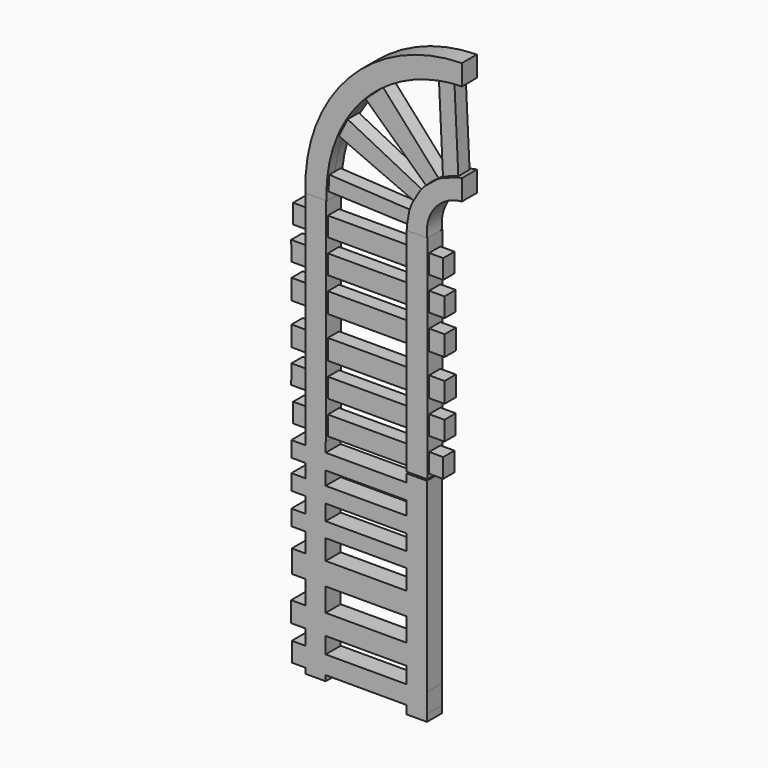
from build123d import *

# Parameters (mm, degrees)
F0_W          = 11.176
F0_H          = 7.62
F0_H_2        = 10.414
F0_H_3        = 10.414198041
F0_H_4        = 10.8981402591
F0_H_5        = 11.3893379234
F0_H_6        = 2.1167141254
F1_DEPTH      = 5.08
F1_DEPTH_BACK = 5.08
F0_W_2        = 43.688
F0_W_3        = 7.62
F0_W_4        = 8.491490941
F0_W_5        = 8.3875925946
F0_W_6        = 8.3293178785
F2_DEPTH      = 3.81
F2_DEPTH_BACK = 3.81
F4_DEPTH      = 5.08
F4_DEPTH_BACK = 5.08
F5_DEPTH      = 3.81
F5_DEPTH_BACK = 3.81
F7_W          = 43.8599754125
F7_H          = 8.4492750466
F7_W_2        = 7.6811425388
F7_H_2        = 8.4492713213
F7_H_3        = 8.4492787719
F7_W_3        = 7.454264909
F7_H_4        = 12.1605284512
F7_W_4        = 7.7864341438
F7_H_5        = 11.0083520412
F7_H_6        = 10.4579478502
F7_H_7        = 9.8724365234
F7_H_8        = 8.0819129944
F8_DEPTH      = 5.08


# Not quite as in the source:
# - a feature names something its author has since deleted; it is built from what else it names


with BuildPart() as f1:
    # F0 (on Front) → F1 (new body, two sides)
    with BuildSketch(Plane.XZ) as f1_sk:
        with Locations((-27.432, 56.4710072617)):
            Rectangle(F0_W, F0_H)
        with Locations((-27.432, 47.4540072617)):
            Rectangle(F0_W, F0_H_2)
        with Locations((-27.432, 38.4370072617)):
            Rectangle(F0_W, F0_H)
        with Locations((-27.432, 29.4199082413)):
            Rectangle(F0_W, F0_H_3)
        with Locations((-27.432, 20.4028092208)):
            Rectangle(F0_W, F0_H)
        with Locations((-27.432, 11.1437390912)):
            Rectangle(F0_W, F0_H_4)
        with Locations((-27.432, 0)):
            Rectangle(F0_W, F0_H_5)
        with Locations((-27.432, -11.1437390912)):
            Rectangle(F0_W, F0_H_4)
        with Locations((-27.432, -20.4028092208)):
            Rectangle(F0_W, F0_H)
        with Locations((-27.432, -29.4199082413)):
            Rectangle(F0_W, F0_H_3)
        with Locations((-27.432, -38.4370072617)):
            Rectangle(F0_W, F0_H)
        with Locations((-27.432, -47.4540072617)):
            Rectangle(F0_W, F0_H_2)
        with Locations((-27.432, -53.7193643245)):
            Rectangle(F0_W, F0_H_6)
    extrude(amount=F1_DEPTH)
    extrude(f1_sk.sketch, amount=-F1_DEPTH_BACK)



with BuildPart() as f1b:
    # F0 (on Front) → F1, piece 2 (new body, two sides)
    with BuildSketch(Plane.XZ) as f1_2_sk:
        with Locations((27.432, -47.4540072617)):
            Rectangle(F0_W, F0_H_2)
        with Locations((27.432, -38.4370072617)):
            Rectangle(F0_W, F0_H)
        with Locations((27.432, -29.4199082413)):
            Rectangle(F0_W, F0_H_3)
        with Locations((27.432, -20.4028092208)):
            Rectangle(F0_W, F0_H)
        with Locations((27.432, -11.1437390912)):
            Rectangle(F0_W, F0_H_4)
        with Locations((27.432, 0)):
            Rectangle(F0_W, F0_H_5)
        with Locations((27.432, 11.1437390912)):
            Rectangle(F0_W, F0_H_4)
        with Locations((27.432, 20.4028092208)):
            Rectangle(F0_W, F0_H)
        with Locations((27.432, 29.4199082413)):
            Rectangle(F0_W, F0_H_3)
        with Locations((27.432, 38.4370072617)):
            Rectangle(F0_W, F0_H)
        with Locations((27.432, 47.4540072617)):
            Rectangle(F0_W, F0_H_2)
        with Locations((27.432, 56.4710072617)):
            Rectangle(F0_W, F0_H)
        with Locations((27.432, -53.7193643245)):
            Rectangle(F0_W, F0_H_6)
    extrude(amount=F1_DEPTH)
    extrude(f1_2_sk.sketch, amount=-F1_DEPTH_BACK)


with BuildPart() as f1_1:
    add(f1.part)

    add(f1b.part)  # F2 merges F1b
    # F0 (on Front) → F2 (join, two sides)
    with BuildSketch(Plane.XZ) as f2_sk:
        with Locations((0, 29.4199082413)):
            Rectangle(F0_W_2, F0_H_3)
        with Locations((0, 47.4540072617)):
            Rectangle(F0_W_2, F0_H_2)
        with Locations((-36.83, 47.4540072617)):
            Rectangle(F0_W_3, F0_H_2)
        Polygon((-33.02, 24.2128092208), (-33.02, 34.6270072617), (-41.7378880084, 34.6270072617), (-41.511490941, 24.2128092208), align=None)
        with Locations((-37.2657454705, 11.1437390912)):
            Rectangle(F0_W_4, F0_H_4)
        with Locations((-37.2657454705, -11.1437390912)):
            Rectangle(F0_W_4, F0_H_4)
        with Locations((0, -11.1437390912)):
            Rectangle(F0_W_2, F0_H_4)
        with Locations((0, 11.1437390912)):
            Rectangle(F0_W_2, F0_H_4)
        with Locations((37.2137962973, -11.1437390912)):
            Rectangle(F0_W_5, F0_H_4)
        with Locations((37.2137962973, 11.1437390912)):
            Rectangle(F0_W_5, F0_H_4)
        with Locations((37.1846589392, 29.4199082413)):
            Rectangle(F0_W_6, F0_H_3)
        with Locations((36.83, 47.4540072617)):
            Rectangle(F0_W_3, F0_H_2)
        with Locations((37.1846589392, -29.4199082413)):
            Rectangle(F0_W_6, F0_H_3)
        with Locations((36.83, -47.4540072617)):
            Rectangle(F0_W_3, F0_H_2)
        with Locations((0, -47.4540072617)):
            Rectangle(F0_W_2, F0_H_2)
        with Locations((0, -29.4199082413)):
            Rectangle(F0_W_2, F0_H_3)
        Polygon((-33.02, -34.6270072617), (-33.02, -24.2128092208), (-41.511490941, -24.2128092208), (-41.7378880084, -34.6270072617), align=None)
        with Locations((-36.83, -47.4540072617)):
            Rectangle(F0_W_3, F0_H_2)
    extrude(amount=F2_DEPTH)
    extrude(f2_sk.sketch, amount=-F2_DEPTH_BACK)

    # F7 (on Front) → F8 (join, symmetric)
    with BuildSketch(Plane.XZ):
        with Locations((-0.098564662, -64.2341207713)):
            Rectangle(F7_W, F7_H)
        Polygon((-22.0285523683, -54.2291179299), (-32.9385772347, -54.2291179299), (-32.9385772347, -60.009483248), (-32.9385772347, -68.4587582946), (-32.9385772347, -75.8059471846), (-32.9385772347, -84.2552185059), (-32.9385772347, -92.7044898272), (-32.9385772347, -101.153768599), (-32.9385772347, -111.6366274655), (-32.9385772347, -123.7971559167), (-32.9385772347, -136.4076882601), (-32.9385772347, -147.4160403013), (-32.9385772347, -155.6722968817), (-32.9385772347, -166.1302447319), (-32.9385772347, -169.044137001), (-22.0285523683, -169.044137001), (-22.0285523683, -166.0951524973), (-22.0285523683, -156.2227159739), (-22.0285523683, -147.4160403013), (-22.0285523683, -136.4076882601), (-22.0285523683, -123.7971559167), (-22.0285523683, -111.6366274655), (-22.0285523683, -100.7864028215), (-22.0285523683, -92.7044898272), (-22.0285523683, -84.2552185059), (-22.0285523683, -75.8059471846), (-22.0285523683, -68.4587582946), (-22.0285523683, -60.009483248), align=None)
        with Locations((-36.7791485041, -64.2341207713)):
            Rectangle(F7_W_2, F7_H)
        with Locations((-36.7791485041, -80.0305828452)):
            Rectangle(F7_W_2, F7_H_2)
        with Locations((-36.7791485041, -96.9291292131)):
            Rectangle(F7_W_2, F7_H_3)
        with Locations((-36.6657096893, -117.7168916911)):
            Rectangle(F7_W_3, F7_H_4)
        with Locations((-36.8317943066, -141.9118642807)):
            Rectangle(F7_W_4, F7_H_5)
        with Locations((-36.6657096893, -160.9012708068)):
            Rectangle(F7_W_3, F7_H_6)
        with Locations((-0.098564662, -161.1589342356)):
            Rectangle(F7_W, F7_H_7)
        with Locations((-0.098564662, -141.9118642807)):
            Rectangle(F7_W, F7_H_5)
        with Locations((-0.098564662, -117.7168916911)):
            Rectangle(F7_W, F7_H_4)
        with Locations((-0.098564662, -96.7454463243)):
            Rectangle(F7_W, F7_H_8)
        with Locations((-0.098564662, -80.0305828452)):
            Rectangle(F7_W, F7_H_2)
        Polygon((21.8314230442, -55.6011721492), (21.8314230442, -60.009483248), (21.8314230442, -68.4587582946), (21.8314230442, -75.8059471846), (21.8314230442, -84.2552185059), (21.8314230442, -92.7044898272), (21.8314230442, -100.7864028215), (21.8314230442, -111.6366274655), (21.8314230442, -123.7971559167), (21.8314230442, -136.4076882601), (21.8314230442, -147.4160403013), (21.8314230442, -156.2227159739), (21.8314230442, -166.0951524973), (21.8314230442, -170.5847382545), (32.8522101045, -170.5847382545), (32.8499992453, -166.8802900054), (32.8436386772, -156.2227159739), (32.7835865319, -55.6011721492), align=None)
    extrude(amount=F8_DEPTH, both=True)


with BuildPart() as f4:
    # F3 (on Front) → F4 (new body, two sides)
    with BuildSketch(Plane.XZ) as f4_sk:
        with BuildLine():
            ThreePointArc((46.7234483179, 138.3806666389), (49.2422027189, 138.5530795685), (51.7653487623, 138.6401657047))
            Line((51.7653487623, 138.6401657047), (51.7653487623, 149.8161657047))
            ThreePointArc((51.7653487623, 149.8161657047), (-9.4395332477, 122.8806362111), (-32.9566933215, 60.2826848626))
            Line((-32.9566933215, 60.2826848626), (-21.428527605, 60.2815099882))
            ThreePointArc((-21.428527605, 60.2815099882), (-21.5025853928, 62.2708854301), (-21.523534037, 64.2615286325))
            ThreePointArc((-21.523534037, 64.2615286325), (-21.4006641675, 68.3361772977), (-21.0554041735, 72.3980308506))
            ThreePointArc((-21.0554041735, 72.3980308506), (-19.1641769465, 82.6655299595), (-15.8580723991, 92.56845635))
            ThreePointArc((-15.8580723991, 92.56845635), (-13.6603359913, 97.3889321711), (-11.1260263684, 102.0412764398))
            ThreePointArc((-11.1260263684, 102.0412764398), (-6.6341482531, 108.7708829528), (-1.4398843374, 114.9744460578))
            ThreePointArc((-1.4398843374, 114.9744460578), (3.1297417642, 119.4636171712), (8.0676414189, 123.5442160236))
            ThreePointArc((8.0676414189, 123.5442160236), (22.4302043573, 132.0660955879), (38.328636759, 137.1793619255))
            ThreePointArc((38.328636759, 137.1793619255), (42.5089587111, 137.8993974077), (46.7234483179, 138.3806666389))
        make_face()
    extrude(amount=F4_DEPTH)
    extrude(f4_sk.sketch, amount=-F4_DEPTH_BACK)



with BuildPart() as f4b:
    # F3 (on Front) → F4, piece 2 (new body, two sides)
    with BuildSketch(Plane.XZ) as f4_2_sk:
        with BuildLine():
            ThreePointArc((33.0161936581, 60.2826066315), (37.2635168322, 76.1212177757), (51.7653487623, 83.7761657047))
            Line((51.7653487623, 83.7761657047), (51.7653487623, 94.9521657047))
            ThreePointArc((51.7653487623, 94.9521657047), (50.2978144115, 94.7028376295), (48.8422158841, 94.3913019379))
            Line((48.8422158841, 94.3913019379), (40.539710538, 91.2735568742))
            ThreePointArc((40.539710538, 91.2735568742), (39.3520349882, 90.6158567529), (38.190774115, 89.9125674487))
            Line((38.190774115, 89.9125674487), (31.4069914905, 84.3135852358))
            ThreePointArc((31.4069914905, 84.3135852358), (30.2440044025, 83.0135126621), (29.1472703966, 81.6570827214))
            Line((29.1472703966, 81.6570827214), (24.9918396341, 74.709399156))
            ThreePointArc((24.9918396341, 74.709399156), (24.0278925704, 72.340750689), (23.2395618841, 69.9080106226))
            Line((23.2395618841, 69.9080106226), (21.9797545722, 62.5895138801))
            ThreePointArc((21.9797545722, 62.5895138801), (21.9248040705, 61.4366528948), (21.9079152744, 60.2826066315))
            Line((21.9079152744, 60.2826066315), (33.0161936581, 60.2826066315))
        make_face()
    extrude(amount=F4_DEPTH)
    extrude(f4_2_sk.sketch, amount=-F4_DEPTH_BACK)


with BuildPart() as f4_1:
    add(f4.part)

    add(f4b.part)  # F5 merges F4b
    # F3 (on Front) → F5 (join, two sides)
    with BuildSketch(Plane.XZ) as f5_sk:
        with BuildLine():
            Line((-21.523534037, 64.2615286325), (21.9797545722, 62.5895138801))
            ThreePointArc((21.9797545722, 62.5895138801), (22.4149059417, 66.2822869441), (23.2395618841, 69.9080106226))
            Line((23.2395618841, 69.9080106226), (-21.0554041735, 72.3980308506))
            Line((-21.0554041735, 72.3980308506), (-21.523534037, 64.2615286325))
        make_face()
        with BuildLine():
            Line((-15.8580723991, 92.56845635), (24.9918396341, 74.709399156))
            ThreePointArc((24.9918396341, 74.709399156), (26.8678964449, 78.3038535456), (29.1472703966, 81.6570827214))
            Line((29.1472703966, 81.6570827214), (-11.1260263684, 102.0412764398))
            Line((-11.1260263684, 102.0412764398), (-15.8580723991, 92.56845635))
        make_face()
        with BuildLine():
            ThreePointArc((31.4069914905, 84.3135852358), (34.6222032412, 87.327143059), (38.190774115, 89.9125674487))
            Line((38.190774115, 89.9125674487), (8.0676414189, 123.5442160236))
            Line((8.0676414189, 123.5442160236), (-1.4398843374, 114.9744460578))
            Line((-1.4398843374, 114.9744460578), (31.4069914905, 84.3135852358))
        make_face()
        with BuildLine():
            ThreePointArc((40.539710538, 91.2735568742), (44.5917613588, 93.0966023555), (48.8422158841, 94.3913019379))
            Line((48.8422158841, 94.3913019379), (46.7234483179, 138.3806666389))
            Line((46.7234483179, 138.3806666389), (38.328636759, 137.1793619255))
            Line((38.328636759, 137.1793619255), (40.539710538, 91.2735568742))
        make_face()
    extrude(amount=F5_DEPTH)
    extrude(f5_sk.sketch, amount=-F5_DEPTH_BACK)


solid = Compound([f1_1.part, f4_1.part])
